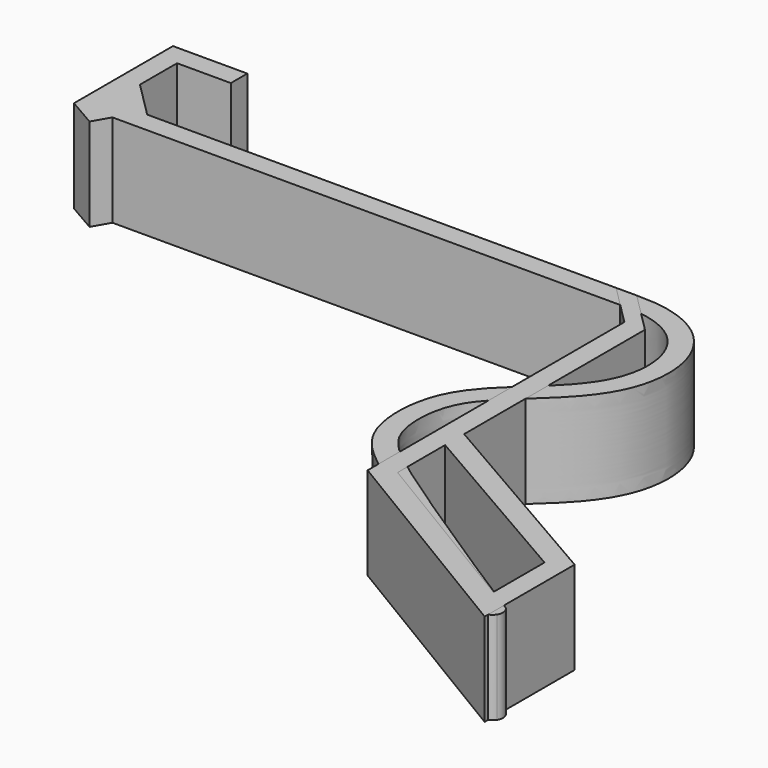
from build123d import *

# Parameters (mm, degrees)
F1_DEPTH     = 9
F3_DEPTH     = 25
F5_DEPTH     = 18
F7_DEPTH     = 18
F8_T1_DEPTH  = 18
F8_T6_DEPTH  = 63.8131565684
F8_T11_DEPTH = 63.8131565684
F11_DEPTH    = 25
F13_DEPTH    = 18
F15_DEPTH    = 25
F17_DEPTH    = 18
F19_DEPTH    = 18
F20_W        = 87.4361209571
F20_H        = 71.8203417063
F21_DEPTH    = 25
F23_DEPTH    = 18
F25_R        = 1.99999


# Not quite as in the source:
# - a fillet or chamfer that OpenCascade refuses, or shapes differently, is made with other operations: its cross-section is extruded or revolved along the edge and cut away or added
# - two fillets or chamfers of one size are made in one step
# - a fillet or chamfer is up to 0.001 mm smaller than in the source, because OpenCascade refuses the exact size
# - the dataset's text gives a spline's control points without its knots; the knots are read off the source's solid


with BuildPart() as f1:
    # F0 (on Top) → F1 (new body, symmetric)
    with BuildSketch(Plane.XY):
        Polygon((-10.432638064, 16), (0, 16), (0, 20), (-14.432638064, 20), (-14.432638064, -4), (91.567361936, -4), (95.567361936, -4), (95.567361936, 0), (-3.432638064, 0), (-10.432638064, 0), (-10.432638064, 7), align=None)
        Polygon((-3.432638064, 0), (-10.432638064, 7), (-10.432638064, 0), align=None)
        Polygon((95.567361936, -4), (91.567361936, -4), (91.567361936, -67.8584948182), (95.567361936, -70.2682493397), align=None)
    extrude(amount=F1_DEPTH, both=True)

    # F2 (on face) → F3 (cut)
    with BuildSketch(Plane.XY.offset(9)):
        Polygon((-43.0447869003, -70.2682493397), (95.567361936, -70.2682493397), (-14.432638064, -4), (-43.0447869003, -4), align=None)
    extrude(amount=-F3_DEPTH, mode=Mode.SUBTRACT)



with BuildPart() as f5:
    # F4 (on face) → F5 (new body)
    with BuildSketch(Plane.XY.offset(9)):
        Polygon((36.264283176, -35.9292474091), (91.567361936, -67.8584948182), (146.870440696, -35.9292474091), (146.870440696, 27.9292474091), (91.567361936, 59.8584948182), (36.264283176, 27.9292474091), align=None)
        Polygon((143.4063390808, -33.9292474091), (91.567361936, -63.8584948182), (39.7283847911, -33.9292474091), (39.7283847911, 25.9292474091), (91.567361936, 55.8584948182), (143.4063390808, 25.9292474091), align=None, mode=Mode.SUBTRACT)
    extrude(amount=-F5_DEPTH)


with BuildPart() as f1_1:
    add(f1.part)

    add(f5.part)  # F7 merges F5
    # F6 (on face) → F7 (join)
    with BuildSketch(Plane.XY.offset(9)):
        Polygon((49.1924864062, -26.7745468707), (95.567361936, -53.5490937415), (141.9422374657, -26.7745468707), (141.9422374657, 26.7745468707), (95.567361936, 53.5490937415), (49.1924864062, 26.7745468707), align=None)
        Polygon((138.4781358506, -24.7745468707), (95.567361936, -49.5490937415), (52.6565880214, -24.7745468707), (52.6565880214, 24.7745468707), (95.567361936, 49.5490937415), (138.4781358506, 24.7745468707), align=None, mode=Mode.SUBTRACT)
    extrude(amount=-F7_DEPTH)

    # F8: chamfer of 8 on 3 edges, made by hand

    # F8_s2 → F8_t1 (cut)
    with BuildSketch(Plane.XY.offset(-9)):
        with BuildLine():
            Line((95.793636106, -8.22627417), (87.341087766, 0.22627417))
            Line((87.341087766, 0.22627417), (87.341087766, 0.38627417))
            ThreePointArc((87.341087766, 0.38627417), (91.454224851, 0.16), (95.567361936, 0.16))
            Line((95.567361936, 0.16), (95.727361936, 0))
            ThreePointArc((95.727361936, 0), (95.727361936, -4.113137085), (95.953636106, -8.22627417))
            Line((95.953636106, -8.22627417), (95.793636106, -8.22627417))
        make_face()
    extrude(amount=F8_T1_DEPTH, mode=Mode.SUBTRACT)


with BuildPart() as f8_tool4:
    # F8_s5 → F8_t6 (new body)
    with BuildSketch(Plane.XZ.offset(4)):
        with BuildLine():
            Line((99.793636106, 9.22627417), (91.341087766, 0.77372583))
            Line((91.341087766, 0.77372583), (91.181087766, 0.77372583))
            ThreePointArc((91.181087766, 0.77372583), (91.407361936, 4.886862915), (91.407361936, 9))
            Line((91.407361936, 9), (91.567361936, 9.16))
            ThreePointArc((91.567361936, 9.16), (95.680499021, 9.16), (99.793636106, 9.38627417))
            Line((99.793636106, 9.38627417), (99.793636106, 9.22627417))
        make_face()
    extrude(amount=F8_T6_DEPTH)

    split(bisect_by=Plane(origin=(2.4364535267, 4.2200612985, 0), x_dir=(0, 0, 1), z_dir=(0.5, 0.8660254038, 0)), keep=Keep.TOP)


with BuildPart() as f1_2:
    add(f1_1.part)

    # F8_t3: cut F8_tool4
    add(f8_tool4.part, mode=Mode.SUBTRACT)


with BuildPart() as f8_tool9:
    # F8_s10 → F8_t11 (new body)
    with BuildSketch(Plane.XZ.offset(4)):
        with BuildLine():
            Line((99.793636106, -9.22627417), (91.341087766, -0.77372583))
            Line((91.341087766, -0.77372583), (91.181087766, -0.77372583))
            ThreePointArc((91.181087766, -0.77372583), (91.407361936, -4.886862915), (91.407361936, -9))
            Line((91.407361936, -9), (91.567361936, -9.16))
            ThreePointArc((91.567361936, -9.16), (95.680499021, -9.16), (99.793636106, -9.38627417))
            Line((99.793636106, -9.38627417), (99.793636106, -9.22627417))
        make_face()
    extrude(amount=F8_T11_DEPTH)

    split(bisect_by=Plane(origin=(2.4364535267, 4.2200612985, 0), x_dir=(0, 0, 1), z_dir=(0.5, 0.8660254038, 0)), keep=Keep.TOP)


with BuildPart() as f1_3:
    add(f1_2.part)

    # F8_t8: cut F8_tool9
    add(f8_tool9.part, mode=Mode.SUBTRACT)

    # F10 (on face) → F11 (cut)
    with BuildSketch(Plane.XY.offset(9)):
        Polygon((24.8906668276, 40.9471578896), (28.4933988005, 0), (95.567361936, 0), (95.567361936, -73.1679201126), (150.7629007101, -38.6447645724), (155.2586406469, 64.3327608705), (108.4874495864, 79.6543508768), align=None)
    extrude(amount=-F11_DEPTH, mode=Mode.SUBTRACT)

    # F12 (on face) → F13 (join)
    with BuildSketch(Plane.XY.offset(9)):
        Polygon((-6.9714882909, -4), (-14.432638064, -4), (-8.8367757342, -7.2307726225), align=None)
    extrude(amount=-F13_DEPTH)

    # F14 (on face) → F15 (cut)
    with BuildSketch(Plane.XY.offset(9)):
        Polygon((95.567361936, -70.2682493397), (-14.432638064, -4), (-31.3558727503, -4), (95.567361936, -79.2363807559), align=None)
    extrude(amount=-F15_DEPTH, mode=Mode.SUBTRACT)

    # F16 (on face) → F17 (join)
    with BuildSketch(Plane.XY.offset(9)):
        Polygon((91.567361936, -67.8584948182), (91.567361936, -63.8584948182), (39.7283847911, -32.6286924278), (36.264283176, -34.5417837953), align=None)
    extrude(amount=-F17_DEPTH)

    # F20 (on face) → F21 (cut)
    with BuildSketch(Plane.XY.offset(9)):
        with Locations((66.817285493, -39.9101708531)):
            Rectangle(F20_W, F20_H)
    extrude(amount=-F21_DEPTH, mode=Mode.SUBTRACT)

    # F22 (on face) → F23 (join)
    with BuildSketch(Plane.XY.offset(9)):
        with BuildLine():
            Line((85.8447179198, 0), (91.567361936, -4))
            add(Edge.make_bspline(
                [(91.567361936, -4), (104.6365553904, -3.7469765326), (110.3428507038, -18.7751399216), (100.6682061408, -31.4519738183), (86.9989600161, -41.7574898726), (86.3592630054, -60.3418471146), (98.3136973624, -70.5662730853), (138.2449475025, -96.0410668665), (139.3067748429, -96.6169106445), (139.4050659721, -96.6777757173)],
                knots=[0, 0, 0, 0, 0.1628326919, 0.297682012, 0.4418751881, 0.5788230188, 0.7291995211, 0.9685112846, 1, 1, 1, 1], degree=3))
            Line((139.4050659721, -96.6777757173), (141.5109392391, -93.2769967208))
            add(Edge.make_bspline(
                [(91.489935257, -0.0007494315), (92.9060638689, 0.026667239), (94.9151446278, -0.0633949156), (97.3780843564, -0.4363427781), (99.1186550622, -0.8406160315), (100.7522644168, -1.3671168497), (102.2764890384, -2.0124833566), (103.687174659, -2.7714731228), (104.9791317233, -3.6362989578), (106.1472476957, -4.5963479152), (107.1877103328, -5.6384829598), (108.0989948056, -6.7478891002), (108.8823349769, -7.9092343833), (109.5416037061, -9.1077354649), (110.2631792919, -10.7375615567), (110.8880990477, -12.8045648004), (111.197246763, -14.8505274464), (111.2848939863, -16.4493183656), (111.2784325522, -17.4284652987), (111.239383264, -18.1975178405), (111.1786575741, -18.9559284858), (111.0629482164, -19.8872137635), (110.8626877911, -20.9765489837), (110.517887814, -22.3889238881), (109.9496817335, -24.075329435), (109.0809935691, -25.9658586266), (108.0601880698, -27.7257624383), (106.9195943398, -29.365227409), (105.6873889524, -30.8991760549), (104.6041921971, -32.1035873015), (103.7142053447, -33.0311278712), (103.1500739634, -33.5975994451), (102.6953807904, -34.0435725593), (102.2398856557, -34.48416563), (101.6695941173, -35.025942992), (100.9869037688, -35.6637824537), (100.0827749646, -36.5005094006), (98.9714726672, -37.5252395865), (97.6913236986, -38.7333149256), (96.4873243456, -39.9292303363), (95.3810591871, -41.119928805), (94.5567517233, -42.111885155), (93.9635091145, -42.9073667468), (93.5530531575, -43.5055894839), (93.2406460512, -44.0061762775), (93.0088635265, -44.408489264), (92.8441318292, -44.7113957423), (92.7145521606, -44.9648366063), (92.6153561916, -45.1686809258), (92.5182097326, -45.3751487314), (92.4010218522, -45.6372959046), (92.2225684087, -46.0652572961), (92.0167949667, -46.6151597501), (91.7982453989, -47.2959410572), (91.6086702998, -47.9943158885), (91.3950994364, -48.9443235243), (91.2023951927, -50.1582211733), (91.0902789156, -51.6272178899), (91.0949751681, -53.0774337202), (91.2115068087, -54.4768084574), (91.3951597463, -55.573143619), (91.5878124211, -56.3912063921), (91.7531885142, -56.9712855308), (91.9364892034, -57.5121789066), (92.1383069402, -58.0194360777), (92.3612623198, -58.502253358), (92.6914841824, -59.1248676607), (93.1774894455, -59.8853754362), (93.9229753903, -60.8261796957), (94.8742532721, -61.8310869152), (96.0631003551, -62.9213330487), (97.5096966069, -64.1125414198), (98.9405899318, -65.2025435375), (100.2252080879, -66.1420739749), (101.2597338638, -66.8830910216), (102.366223827, -67.6629682078), (103.5464743012, -68.4851737705), (104.7925271914, -69.3451211004), (106.0977962495, -70.2385676403), (107.4556943956, -71.1614354801), (109.327763763, -72.425777016), (111.7671477763, -74.0596996937), (114.8023314083, -76.0744652395), (118.9257582498, -78.7912727197), (123.0632736591, -81.4916101611), (127.0143083715, -84.0517644681), (129.8343013517, -85.8709345559), (132.4609442879, -87.5582903798), (134.8441158986, -89.0829323591), (136.9335516879, -90.413872351), (138.6784873332, -91.5198131291), (139.8024005469, -92.2273441725), (140.3905760047, -92.5946857153), (140.6306590714, -92.7436984022), (140.7515869067, -92.8184414331), (140.8610086419, -92.8858419225), (140.9773867305, -92.9570703604), (141.088989496, -93.0247655444), (141.1764306926, -93.0772952846), (141.2449004889, -93.1180398404), (141.3013989116, -93.1514059016), (141.3559414676, -93.1835286385), (141.4214007655, -93.2223160073), (141.479103077, -93.2572827309), (141.5109392391, -93.2769967208)],
                knots=[0, 0, 0, 0, 0.015625, 0.0234375, 0.03125, 0.0390625, 0.046875, 0.0546875, 0.0625, 0.0703125, 0.078125, 0.0859375, 0.09375, 0.1015625, 0.109375, 0.125, 0.140625, 0.1484375, 0.15625, 0.16015625, 0.1640625, 0.171875, 0.1796875, 0.1875, 0.203125, 0.21875, 0.234375, 0.25, 0.265625, 0.28125, 0.2890625, 0.296875, 0.30078125, 0.3046875, 0.3125, 0.3203125, 0.328125, 0.34375, 0.359375, 0.375, 0.390625, 0.40625, 0.4140625, 0.421875, 0.4296875, 0.43359375, 0.4375, 0.44140625, 0.443359375, 0.4453125, 0.44921875, 0.453125, 0.4609375, 0.46875, 0.4765625, 0.484375, 0.5, 0.515625, 0.53125, 0.546875, 0.5625, 0.5703125, 0.578125, 0.5859375, 0.59375, 0.6015625, 0.609375, 0.625, 0.640625, 0.65625, 0.671875, 0.6875, 0.703125, 0.7109375, 0.71875, 0.7265625, 0.734375, 0.7421875, 0.75, 0.7578125, 0.765625, 0.78125, 0.796875, 0.8125, 0.84375, 0.859375, 0.875, 0.890625, 0.90625, 0.921875, 0.9375, 0.953125, 0.9609375, 0.96484375, 0.966796875, 0.96875, 0.97265625, 0.9765625, 0.98046875, 0.984375, 0.98828125, 0.9921875, 0.99609375, 1, 1, 1, 1], degree=3))
            Line((91.489935257, -0.0007494315), (85.8447179198, 0))
        make_face()
    extrude(amount=-F23_DEPTH)

    # F25 (radius 2 in the source; OpenCascade refuses exactly that, so slightly less here)
    f25_edges = [f1_3.edges().sort_by_distance(p)[0] for p in [
        (139.405066, -96.677776, 0),
        (141.510939, -93.276997, 0),
    ]]
    fillet(f25_edges, radius=F25_R)


with BuildPart() as f19:
    # F18 (on face) → F19 (new body)
    with BuildSketch(Plane.XY.offset(9)):
        Polygon((95.567361936, -65.5984616728), (95.567361936, -70.2682493397), (139.4050659721, -96.6777757173), (139.4050659721, -92.0079880504), (135.4050659721, -89.598233529), (99.567361936, -68.0082161942), align=None)
        Polygon((95.567361936, -54.167895895), (95.567361936, -65.5984616728), (99.567361936, -68.0082161942), (99.567361936, -56.4772969717), align=None)
        Polygon((135.4050659721, -89.598233529), (139.4050659721, -92.0079880504), (139.4050659721, -79.4776061209), (135.4050659721, -77.1682050441), align=None)
        Polygon((95.567361936, -49.5490937415), (95.567361936, -54.167895895), (99.567361936, -56.4772969717), (99.567361936, -51.8584948182), align=None)
        Polygon((135.4050659721, -77.1682050441), (139.4050659721, -79.4776061209), (139.4050659721, -74.8588039673), (131.4809072449, -70.2837887931), (99.567361936, -51.8584948182), (99.567361936, -56.4772969717), align=None)
        Polygon((95.567361936, -8), (95.567361936, -49.5490937415), (99.567361936, -51.8584948182), (99.567361936, -8), (91.567361936, 0), (87.567361936, 0), align=None)
    extrude(amount=-F19_DEPTH)


solid = Compound([f1_3.part, f19.part])
